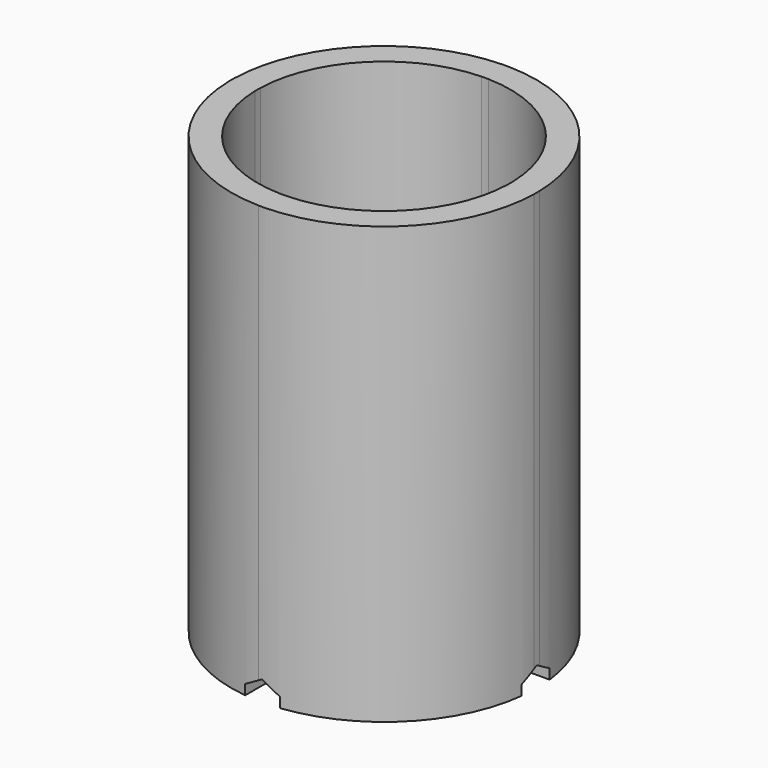
from build123d import *

# Parameters (mm, degrees)
F0_W     = 1.6
F0_H     = 1.6
F0_H_2   = 11.3644893661
F0_W_2   = 11.3644893661
F1_DEPTH = 10
F2_DEPTH = 100
F4_DEPTH = 100
F6_DEPTH = 100
F7_DEPTH = 0.01


# Not quite as in the source:
# - a feature of the source that left no trace in its solid (it failed there, or was rolled back) is left out
# - a feature names something its author has since deleted; it is built from what else it names


with BuildPart() as f1:
    # F0 (on Top) → F1 (new body)
    with BuildSketch(Plane.XY):
        with BuildLine():
            Line((-0.8, 34.9908559484), (0.8, 34.9908559484))
            ThreePointArc((0.8, 34.9908559484), (0, 35), (-0.8, 34.9908559484))
        make_face()
        with BuildLine():
            Line((-34.9908559484, -0.8), (-34.9908559484, 0.8))
            ThreePointArc((-34.9908559484, 0.8), (-35, 0), (-34.9908559484, -0.8))
        make_face()
        with BuildLine():
            ThreePointArc((-0.8, -34.9908559484), (0, -35), (0.8, -34.9908559484))
            Line((0.8, -34.9908559484), (-0.8, -34.9908559484))
        make_face()
        with BuildLine():
            ThreePointArc((34.9908559484, -0.8), (34.9977139124, -0.4000261284), (35, 0))
            ThreePointArc((35, 0), (34.9977139124, 0.4000261284), (34.9908559484, 0.8))
            Line((34.9908559484, 0.8), (34.9908559484, -0.8))
        make_face()
        with BuildLine():
            Line((28.9889634171, 0.8), (34.9908559484, 0.8))
            ThreePointArc((34.9908559484, 0.8), (24.7487373415, 24.7487373415), (0.8, 34.9908559484))
            Line((0.8, 34.9908559484), (0.8, 28.9889634171))
            ThreePointArc((0.8, 28.9889634171), (20.5060966544, 20.5060966544), (28.9889634171, 0.8))
        make_face()
        with BuildLine():
            ThreePointArc((-34.9908559484, -0.8), (-24.7487373415, -24.7487373415), (-0.8, -34.9908559484))
            Line((-0.8, -34.9908559484), (-0.8, -28.9889634171))
            ThreePointArc((-0.8, -28.9889634171), (-20.5060966544, -20.5060966544), (-28.9889634171, -0.8))
            Line((-28.9889634171, -0.8), (-34.9908559484, -0.8))
        make_face()
        with BuildLine():
            ThreePointArc((0.8, -34.9908559484), (24.7487373415, -24.7487373415), (34.9908559484, -0.8))
            Line((34.9908559484, -0.8), (28.9889634171, -0.8))
            ThreePointArc((28.9889634171, -0.8), (20.5060966544, -20.5060966544), (0.8, -28.9889634171))
            Line((0.8, -28.9889634171), (0.8, -34.9908559484))
        make_face()
        with BuildLine():
            Line((0.8, 28.9889634171), (0.8, 34.9908559484))
            Line((0.8, 34.9908559484), (-0.8, 34.9908559484))
            Line((-0.8, 34.9908559484), (-0.8, 28.9889634171))
            ThreePointArc((-0.8, 28.9889634171), (0, 29), (0.8, 28.9889634171))
        make_face()
        with BuildLine():
            Line((-28.9889634171, 0.8), (-34.9908559484, 0.8))
            Line((-34.9908559484, 0.8), (-34.9908559484, -0.8))
            Line((-34.9908559484, -0.8), (-28.9889634171, -0.8))
            ThreePointArc((-28.9889634171, -0.8), (-29, 0), (-28.9889634171, 0.8))
        make_face()
        with BuildLine():
            Line((-0.8, -34.9908559484), (0.8, -34.9908559484))
            Line((0.8, -34.9908559484), (0.8, -28.9889634171))
            ThreePointArc((0.8, -28.9889634171), (0, -29), (-0.8, -28.9889634171))
            Line((-0.8, -28.9889634171), (-0.8, -34.9908559484))
        make_face()
        with BuildLine():
            Line((34.9908559484, -0.8), (34.9908559484, 0.8))
            Line((34.9908559484, 0.8), (28.9889634171, 0.8))
            ThreePointArc((28.9889634171, 0.8), (28.997240723, 0.4000380626), (29, 0))
            ThreePointArc((29, 0), (28.997240723, -0.4000380626), (28.9889634171, -0.8))
            Line((28.9889634171, -0.8), (34.9908559484, -0.8))
        make_face()
        with BuildLine():
            Line((-0.8, 12.1644893661), (-0.8, 28.9889634171))
            ThreePointArc((-0.8, 28.9889634171), (-20.5060966544, 20.5060966544), (-28.9889634171, 0.8))
            Line((-28.9889634171, 0.8), (-12.1644893661, 0.8))
            Line((-12.1644893661, 0.8), (-12.1644893661, 3.259465102))
            Line((-12.1644893661, 3.259465102), (-8.9050242641, 8.9050242641))
            Line((-8.9050242641, 8.9050242641), (-3.259465102, 12.1644893661))
            Line((-3.259465102, 12.1644893661), (-0.8, 12.1644893661))
        make_face()
        with BuildLine():
            Line((-0.8, 28.9889634171), (-0.8, 34.9908559484))
            ThreePointArc((-0.8, 34.9908559484), (-24.7487373415, 24.7487373415), (-34.9908559484, 0.8))
            Line((-34.9908559484, 0.8), (-28.9889634171, 0.8))
            ThreePointArc((-28.9889634171, 0.8), (-20.5060966544, 20.5060966544), (-0.8, 28.9889634171))
        make_face()
        with BuildLine():
            Line((-12.1644893661, 0.8), (-28.9889634171, 0.8))
            ThreePointArc((-28.9889634171, 0.8), (-29, 0), (-28.9889634171, -0.8))
            Line((-28.9889634171, -0.8), (-12.1644893661, -0.8))
            Line((-12.1644893661, -0.8), (-12.1644893661, 0.8))
        make_face()
        with BuildLine():
            ThreePointArc((-28.9889634171, -0.8), (-20.5060966544, -20.5060966544), (-0.8, -28.9889634171))
            Line((-0.8, -28.9889634171), (-0.8, -12.1644893661))
            Line((-0.8, -12.1644893661), (-3.259465102, -12.1644893661))
            Line((-3.259465102, -12.1644893661), (-8.9050242641, -8.9050242641))
            Line((-8.9050242641, -8.9050242641), (-12.1644893661, -3.259465102))
            Line((-12.1644893661, -3.259465102), (-12.1644893661, -0.8))
            Line((-12.1644893661, -0.8), (-28.9889634171, -0.8))
        make_face()
        with BuildLine():
            ThreePointArc((-0.8, -28.9889634171), (0, -29), (0.8, -28.9889634171))
            Line((0.8, -28.9889634171), (0.8, -12.1644893661))
            Line((0.8, -12.1644893661), (-0.8, -12.1644893661))
            Line((-0.8, -12.1644893661), (-0.8, -28.9889634171))
        make_face()
        with BuildLine():
            ThreePointArc((29, 0), (28.997240723, 0.4000380626), (28.9889634171, 0.8))
            Line((28.9889634171, 0.8), (12.1644893661, 0.8))
            Line((12.1644893661, 0.8), (12.1644893661, -0.8))
            Line((12.1644893661, -0.8), (28.9889634171, -0.8))
            ThreePointArc((28.9889634171, -0.8), (28.997240723, -0.4000380626), (29, 0))
        make_face()
        Rectangle(F0_W, F0_H)
        with BuildLine():
            Line((0.8, 12.1644893661), (0.8, 28.9889634171))
            ThreePointArc((0.8, 28.9889634171), (0, 29), (-0.8, 28.9889634171))
            Line((-0.8, 28.9889634171), (-0.8, 12.1644893661))
            Line((-0.8, 12.1644893661), (0.8, 12.1644893661))
        make_face()
        with BuildLine():
            Line((12.1644893661, 0.8), (28.9889634171, 0.8))
            ThreePointArc((28.9889634171, 0.8), (20.5060966544, 20.5060966544), (0.8, 28.9889634171))
            Line((0.8, 28.9889634171), (0.8, 12.1644893661))
            Line((0.8, 12.1644893661), (3.259465102, 12.1644893661))
            Line((3.259465102, 12.1644893661), (8.9050242641, 8.9050242641))
            Line((8.9050242641, 8.9050242641), (12.1644893661, 3.259465102))
            Line((12.1644893661, 3.259465102), (12.1644893661, 0.8))
        make_face()
        with BuildLine():
            ThreePointArc((0.8, -28.9889634171), (20.5060966544, -20.5060966544), (28.9889634171, -0.8))
            Line((28.9889634171, -0.8), (12.1644893661, -0.8))
            Line((12.1644893661, -0.8), (12.1644893661, -3.259465102))
            Line((12.1644893661, -3.259465102), (8.9050242641, -8.9050242641))
            Line((8.9050242641, -8.9050242641), (3.259465102, -12.1644893661))
            Line((3.259465102, -12.1644893661), (0.8, -12.1644893661))
            Line((0.8, -12.1644893661), (0.8, -28.9889634171))
        make_face()
        Polygon((-0.8, 0.8), (-0.8, 12.1644893661), (-3.259465102, 12.1644893661), (-8.9050242641, 8.9050242641), (-12.1644893661, 3.259465102), (-12.1644893661, 0.8), align=None)
        Polygon((-3.259465102, -12.1644893661), (-0.8, -12.1644893661), (-0.8, -0.8), (-12.1644893661, -0.8), (-12.1644893661, -3.259465102), (-8.9050242641, -8.9050242641), align=None)
        Polygon((12.1644893661, -3.259465102), (12.1644893661, -0.8), (0.8, -0.8), (0.8, -12.1644893661), (3.259465102, -12.1644893661), (8.9050242641, -8.9050242641), align=None)
        Polygon((0.8, 0.8), (12.1644893661, 0.8), (12.1644893661, 3.259465102), (8.9050242641, 8.9050242641), (3.259465102, 12.1644893661), (0.8, 12.1644893661), align=None)
        with Locations((0, 6.4822446831)):
            Rectangle(F0_W, F0_H_2)
        with Locations((-6.4822446831, 0)):
            Rectangle(F0_W_2, F0_H)
        with Locations((0, -6.4822446831)):
            Rectangle(F0_W, F0_H_2)
        with Locations((6.4822446831, 0)):
            Rectangle(F0_W_2, F0_H)
    extrude(amount=F1_DEPTH)

    # F0 (on Top) → F2 (join)
    with BuildSketch(Plane.XY):
        with BuildLine():
            ThreePointArc((34.9908559484, -0.8), (34.9977139124, -0.4000261284), (35, 0))
            ThreePointArc((35, 0), (34.9977139124, 0.4000261284), (34.9908559484, 0.8))
            Line((34.9908559484, 0.8), (34.9908559484, -0.8))
        make_face()
        with BuildLine():
            Line((28.9889634171, 0.8), (34.9908559484, 0.8))
            ThreePointArc((34.9908559484, 0.8), (24.7487373415, 24.7487373415), (0.8, 34.9908559484))
            Line((0.8, 34.9908559484), (0.8, 28.9889634171))
            ThreePointArc((0.8, 28.9889634171), (20.5060966544, 20.5060966544), (28.9889634171, 0.8))
        make_face()
        with BuildLine():
            Line((34.9908559484, -0.8), (34.9908559484, 0.8))
            Line((34.9908559484, 0.8), (28.9889634171, 0.8))
            ThreePointArc((28.9889634171, 0.8), (28.997240723, 0.4000380626), (29, 0))
            ThreePointArc((29, 0), (28.997240723, -0.4000380626), (28.9889634171, -0.8))
            Line((28.9889634171, -0.8), (34.9908559484, -0.8))
        make_face()
        with BuildLine():
            ThreePointArc((0.8, -34.9908559484), (24.7487373415, -24.7487373415), (34.9908559484, -0.8))
            Line((34.9908559484, -0.8), (28.9889634171, -0.8))
            ThreePointArc((28.9889634171, -0.8), (20.5060966544, -20.5060966544), (0.8, -28.9889634171))
            Line((0.8, -28.9889634171), (0.8, -34.9908559484))
        make_face()
        with BuildLine():
            Line((-0.8, 34.9908559484), (0.8, 34.9908559484))
            ThreePointArc((0.8, 34.9908559484), (0, 35), (-0.8, 34.9908559484))
        make_face()
        with BuildLine():
            Line((0.8, 28.9889634171), (0.8, 34.9908559484))
            Line((0.8, 34.9908559484), (-0.8, 34.9908559484))
            Line((-0.8, 34.9908559484), (-0.8, 28.9889634171))
            ThreePointArc((-0.8, 28.9889634171), (0, 29), (0.8, 28.9889634171))
        make_face()
        with BuildLine():
            ThreePointArc((-0.8, -34.9908559484), (0, -35), (0.8, -34.9908559484))
            Line((0.8, -34.9908559484), (-0.8, -34.9908559484))
        make_face()
        with BuildLine():
            Line((-0.8, -34.9908559484), (0.8, -34.9908559484))
            Line((0.8, -34.9908559484), (0.8, -28.9889634171))
            ThreePointArc((0.8, -28.9889634171), (0, -29), (-0.8, -28.9889634171))
            Line((-0.8, -28.9889634171), (-0.8, -34.9908559484))
        make_face()
        with BuildLine():
            Line((-0.8, 28.9889634171), (-0.8, 34.9908559484))
            ThreePointArc((-0.8, 34.9908559484), (-24.7487373415, 24.7487373415), (-34.9908559484, 0.8))
            Line((-34.9908559484, 0.8), (-28.9889634171, 0.8))
            ThreePointArc((-28.9889634171, 0.8), (-20.5060966544, 20.5060966544), (-0.8, 28.9889634171))
        make_face()
        with BuildLine():
            ThreePointArc((-34.9908559484, -0.8), (-24.7487373415, -24.7487373415), (-0.8, -34.9908559484))
            Line((-0.8, -34.9908559484), (-0.8, -28.9889634171))
            ThreePointArc((-0.8, -28.9889634171), (-20.5060966544, -20.5060966544), (-28.9889634171, -0.8))
            Line((-28.9889634171, -0.8), (-34.9908559484, -0.8))
        make_face()
        with BuildLine():
            Line((-34.9908559484, -0.8), (-34.9908559484, 0.8))
            ThreePointArc((-34.9908559484, 0.8), (-35, 0), (-34.9908559484, -0.8))
        make_face()
        with BuildLine():
            Line((-28.9889634171, 0.8), (-34.9908559484, 0.8))
            Line((-34.9908559484, 0.8), (-34.9908559484, -0.8))
            Line((-34.9908559484, -0.8), (-28.9889634171, -0.8))
            ThreePointArc((-28.9889634171, -0.8), (-29, 0), (-28.9889634171, 0.8))
        make_face()
    extrude(amount=F2_DEPTH)

    # F3 (on Front) → F4 (cut, symmetric)
    with BuildSketch(Plane.XZ):
        Polygon((4, -2.3094010768), (4, 2.3094010768), (0, 4.6188021535), (-4, 2.3094010768), (-4, -2.3094010768), (0, -4.6188021535), align=None)
    extrude(amount=F4_DEPTH, both=True, mode=Mode.SUBTRACT)

    # F5 (on Right) → F6 (cut, symmetric)
    with BuildSketch(Plane.YZ):
        Polygon((-4, 2.3094010768), (-4, -2.3094010768), (0, -4.6188021535), (4, -2.3094010768), (4, 2.3094010768), (0, 4.6188021535), align=None)
    extrude(amount=F6_DEPTH, both=True, mode=Mode.SUBTRACT)


with BuildPart() as f7:
    # F0 (on Top) → F7 (new body)
    with BuildSketch(Plane.XY):
        Polygon((-3.259465102, -12.1644893661), (-0.8, -12.1644893661), (-0.8, -0.8), (-12.1644893661, -0.8), (-12.1644893661, -3.259465102), (-8.9050242641, -8.9050242641), align=None)
        Polygon((12.1644893661, -3.259465102), (12.1644893661, -0.8), (0.8, -0.8), (0.8, -12.1644893661), (3.259465102, -12.1644893661), (8.9050242641, -8.9050242641), align=None)
        Polygon((0.8, 0.8), (12.1644893661, 0.8), (12.1644893661, 3.259465102), (8.9050242641, 8.9050242641), (3.259465102, 12.1644893661), (0.8, 12.1644893661), align=None)
        Polygon((-0.8, 0.8), (-0.8, 12.1644893661), (-3.259465102, 12.1644893661), (-8.9050242641, 8.9050242641), (-12.1644893661, 3.259465102), (-12.1644893661, 0.8), align=None)
        with Locations((-6.4822446831, 0)):
            Rectangle(F0_W_2, F0_H)
        with Locations((6.4822446831, 0)):
            Rectangle(F0_W_2, F0_H)
        with Locations((0, 6.4822446831)):
            Rectangle(F0_W, F0_H_2)
        with Locations((0, -6.4822446831)):
            Rectangle(F0_W, F0_H_2)
    extrude(amount=F7_DEPTH)


solid = Compound([f1.part, f7.part])
